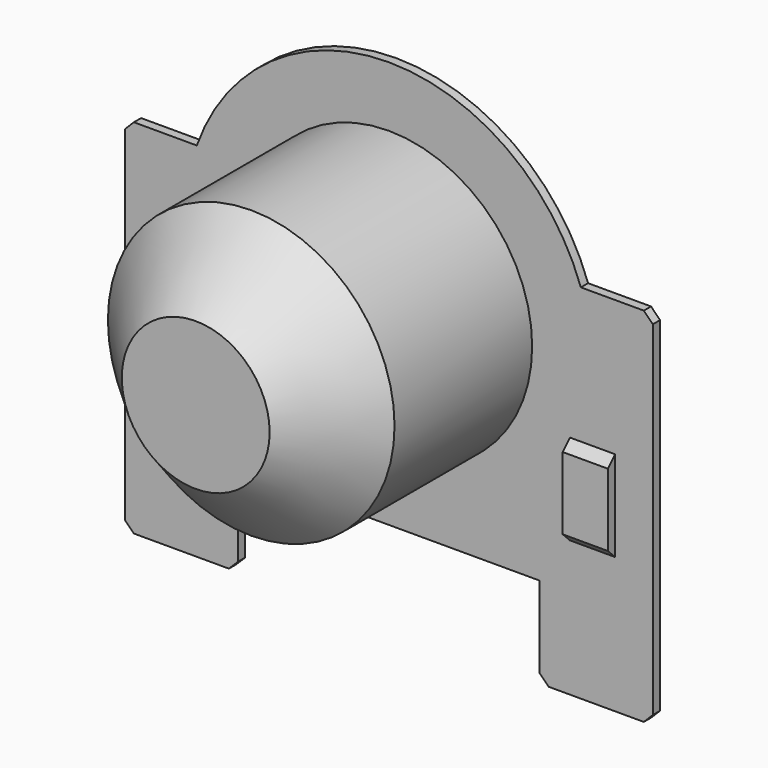
from build123d import *

# Parameters (mm, degrees)
F0_W     = 1.5
F0_H     = 3
F1_DEPTH = 0.3
F2_DEPTH = 0.6
F3_R     = 4.75
F4_DEPTH = 8
F5_SIZE  = 2.3
F6_SIZE  = 0.29999


# Not quite as in the source:
# - a fillet or chamfer is up to 0.001 mm smaller than in the source, because OpenCascade refuses the exact size


with BuildPart() as f1:
    # F0 (on Front) → F1 (new body)
    with BuildSketch(Plane.XZ):
        with BuildLine():
            Line((8.75, -6), (8.75, 6))
            Line((8.75, 6), (6.3639610307, 6))
            ThreePointArc((6.3639610307, 6), (0, 10.5), (-6.3639610307, 6))
            Line((-6.3639610307, 6), (-8.75, 6))
            Line((-8.75, 6), (-8.75, -6))
            Line((-8.75, -6), (-5, -6))
            Line((-5, -6), (-5, -3))
            Line((-5, -3), (5, -3))
            Line((5, -3), (5, -6))
            Line((5, -6), (8.75, -6))
        make_face()
        with Locations((-6.75, 0)):
            Rectangle(F0_W, F0_H, mode=Mode.SUBTRACT)
        with Locations((6.75, 0)):
            Rectangle(F0_W, F0_H, mode=Mode.SUBTRACT)
        with Locations((-6.75, 0)):
            Rectangle(F0_W, F0_H)
        with Locations((6.75, 0)):
            Rectangle(F0_W, F0_H)
    extrude(amount=F1_DEPTH)

    # F0 (on Front) → F2 (join)
    with BuildSketch(Plane.XZ):
        with Locations((-6.75, 0)):
            Rectangle(F0_W, F0_H)
        with Locations((6.75, 0)):
            Rectangle(F0_W, F0_H)
    extrude(amount=F2_DEPTH)

    # F3 (on face) → F4 (join)
    with BuildSketch(Plane.XZ.offset(0.3)):
        with Locations((0, 3.75)):
            Circle(F3_R)
    extrude(amount=F4_DEPTH)

    # F5
    f5_edges = [f1.edges().sort_by_distance(p)[0] for p in [
        (-4.75, -8.3, 3.75),
    ]]
    chamfer(f5_edges, length=F5_SIZE)

    # F6 (size 0.3 in the source; OpenCascade refuses exactly that, so slightly less here)
    f6_edges = [f1.edges().sort_by_distance(p)[0] for p in [
        (-6.75, -0.6, -1.5),
        (-6.75, -0.6, 1.5),
        (6.75, -0.6, -1.5),
        (6.75, -0.6, 1.5),
        (-5, -0.15, -6),
        (-8.75, -0.15, -6),
        (5, -0.15, -6),
        (8.75, -0.15, -6),
        (8.75, -0.15, 6),
        (-8.75, -0.15, 6),
    ]]
    chamfer(f6_edges, length=F6_SIZE)


solid = f1.part
